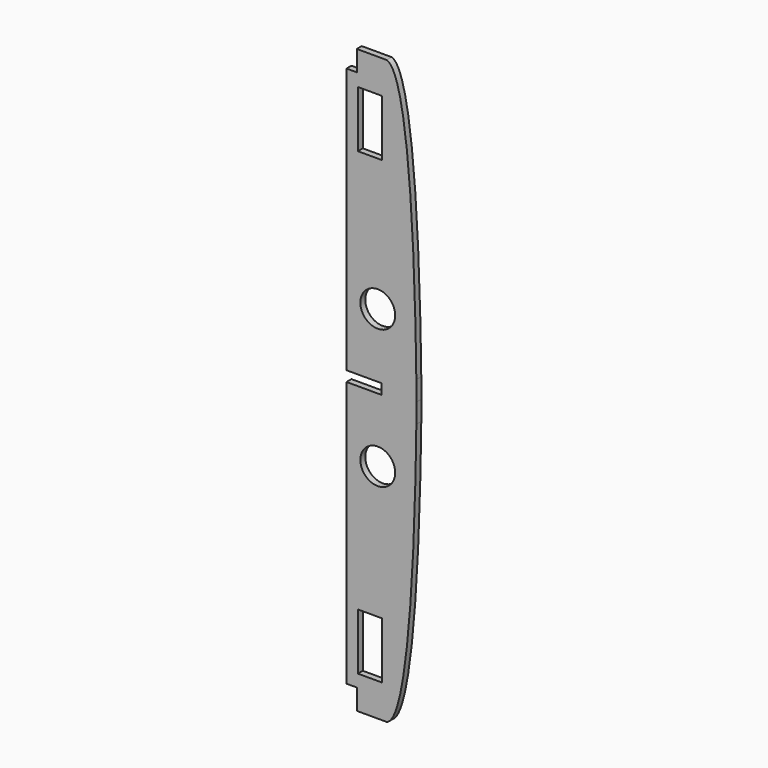
from build123d import *

# Parameters (mm, degrees)
F0_W     = 23.2594013214
F0_H     = 54.8999868333
F0_R     = 16.9272487263
F1_DEPTH = 6


# Not quite as in the source:
# - a feature names something its author has since deleted; it is built from what else it names


with BuildPart() as f1:
    # F0 (on Front) → F1 (new body)
    with BuildSketch(Plane.XZ):
        with BuildLine():
            add(Edge.make_bspline(
                [(266.3061527885, -172.8736048774), (266.4418306907, -161.1180388855), (266.4673413702, -154.0153294904), (266.4976486654, -153.6832076827)],
                knots=[239.4581463651, 239.4581463651, 239.4581463651, 239.4581463651, 284.4819853699, 284.4819853699, 284.4819853699, 284.4819853699], degree=3))
            Line((266.4976486654, -153.6832076827), (232.4976486654, -153.6832076827))
            Line((232.4976486654, -153.6832076827), (232.4976486654, -158.6832076827))
            Line((232.4976486654, -158.6832076827), (198.4976486654, -158.6832076827))
            Line((198.4976486654, -158.6832076827), (198.4976486654, -416.6832076827))
            Line((198.4976486654, -416.6832076827), (208.4976486654, -416.6832076827))
            Line((208.4976486654, -416.6832076827), (208.4976486654, -436.6832076827))
            Line((208.4976486654, -436.6832076827), (237.4976486654, -436.6832076827))
            add(Edge.make_bspline(
                [(237.4976486654, -436.6832076827), (261.7467447475, -429.5284690744), (265.5845533054, -235.3952845947), (266.3061527885, -172.8736048774)],
                knots=[0, 0, 0, 0, 239.4581463651, 239.4581463651, 239.4581463651, 239.4581463651], degree=3))
        make_face()
        with Locations((221.1196951035, -377.0302243151)):
            Rectangle(F0_W, F0_H, mode=Mode.SUBTRACT)
        with Locations((228.8340181112, -220.9526370094)):
            Circle(F0_R, mode=Mode.SUBTRACT)
        with BuildLine():
            add(Edge.make_bspline(
                [(237.4976486654, 129.3167923173), (261.7467447475, 122.1620537089), (265.5845533054, -71.9711307708), (266.3061527885, -134.492810488)],
                knots=[0, 0, 0, 0, 239.4581463651, 239.4581463651, 239.4581463651, 239.4581463651], degree=3))
            Line((237.4976486654, 129.3167923173), (208.4976486654, 129.3167923173))
            Line((208.4976486654, 129.3167923173), (208.4976486654, 109.3167923173))
            Line((208.4976486654, 109.3167923173), (198.4976486654, 109.3167923173))
            Line((198.4976486654, 109.3167923173), (198.4976486654, -148.6832076827))
            Line((198.4976486654, -148.6832076827), (232.4976486654, -148.6832076827))
            Line((232.4976486654, -148.6832076827), (232.4976486654, -153.6832076827))
            Line((232.4976486654, -153.6832076827), (266.4976486654, -153.6832076827))
            add(Edge.make_bspline(
                [(266.3061527885, -134.492810488), (266.4418306907, -146.24837648), (266.4673413702, -153.3510858751), (266.4976486654, -153.6832076827)],
                knots=[239.4581463651, 239.4581463651, 239.4581463651, 239.4581463651, 284.4819853699, 284.4819853699, 284.4819853699, 284.4819853699], degree=3))
        make_face()
        with Locations((228.8340181112, -86.4137783561)):
            Circle(F0_R, mode=Mode.SUBTRACT)
        with Locations((221.1196951035, 69.6638089497)):
            Rectangle(F0_W, F0_H, mode=Mode.SUBTRACT)
    extrude(amount=F1_DEPTH)


solid = f1.part
